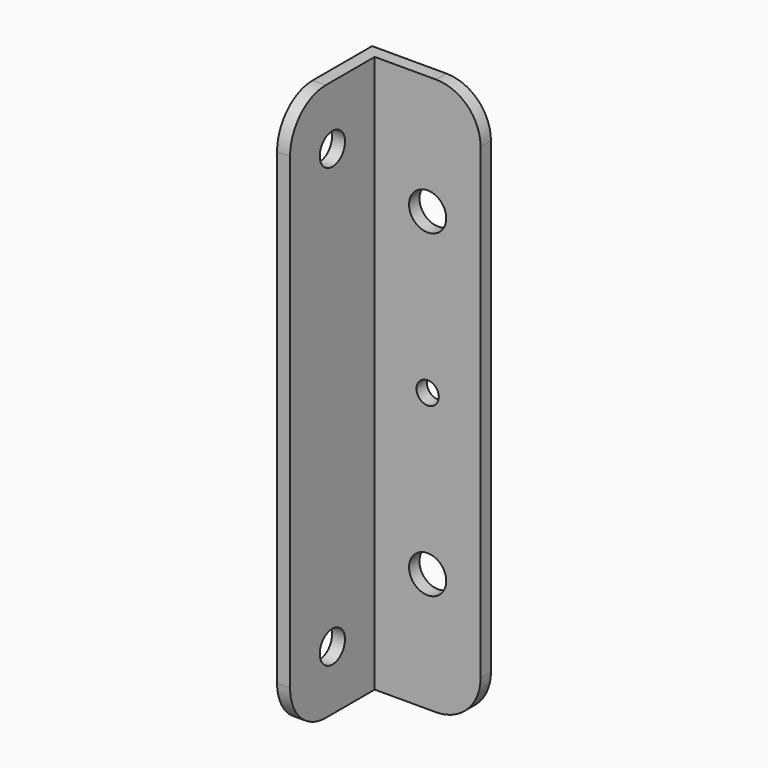
from build123d import *

# Parameters (mm, degrees)
F1_DEPTH = 150
F3_D     = 8.5
F3_DEPTH = 16.5
F3_TIP   = 2.5536576309
F5_D     = 10
F5_DEPTH = 25
F5_TIP   = 3.0043030951
F7_D     = 6
F7_DEPTH = 25
F7_TIP   = 1.8025818571
F8_R     = 12


with BuildPart() as f1:
    # F0 (on Top) → F1 (new body)
    with BuildSketch(Plane.XY):
        Polygon((32, -3.5), (32, 0), (0, 0), (0, -32), (3.5, -32), (3.5, -3.5), align=None)
    extrude(amount=F1_DEPTH)

    # F3
    with Locations(Plane.YZ.offset(3.5)):
        with Locations((-17.75, 134), (-17.75, 16)):
            Hole(F3_D / 2, depth=F3_DEPTH)
            with Locations((0, 0, -(F3_DEPTH + F3_TIP / 2))):  # 118° drill point
                Cone(0, F3_D / 2, F3_TIP, mode=Mode.SUBTRACT)

    # F5
    with Locations(Plane.XZ.offset(3.5)):
        with Locations((17.75, 118), (17.75, 32)):
            Hole(F5_D / 2, depth=F5_DEPTH)
            with Locations((0, 0, -(F5_DEPTH + F5_TIP / 2))):  # 118° drill point
                Cone(0, F5_D / 2, F5_TIP, mode=Mode.SUBTRACT)

    # F7
    with Locations(Plane.XZ.offset(3.5)):
        with Locations((17.75, 75)):
            Hole(F7_D / 2, depth=F7_DEPTH)
            with Locations((0, 0, -(F7_DEPTH + F7_TIP / 2))):  # 118° drill point
                Cone(0, F7_D / 2, F7_TIP, mode=Mode.SUBTRACT)

    # F8
    f8_edges = [f1.edges().sort_by_distance(p)[0] for p in [
        (1.75, -32, 150),
        (32, -1.75, 150),
        (32, -1.75, 0),
        (1.75, -32, 0),
    ]]
    fillet(f8_edges, radius=F8_R)


solid = f1.part
